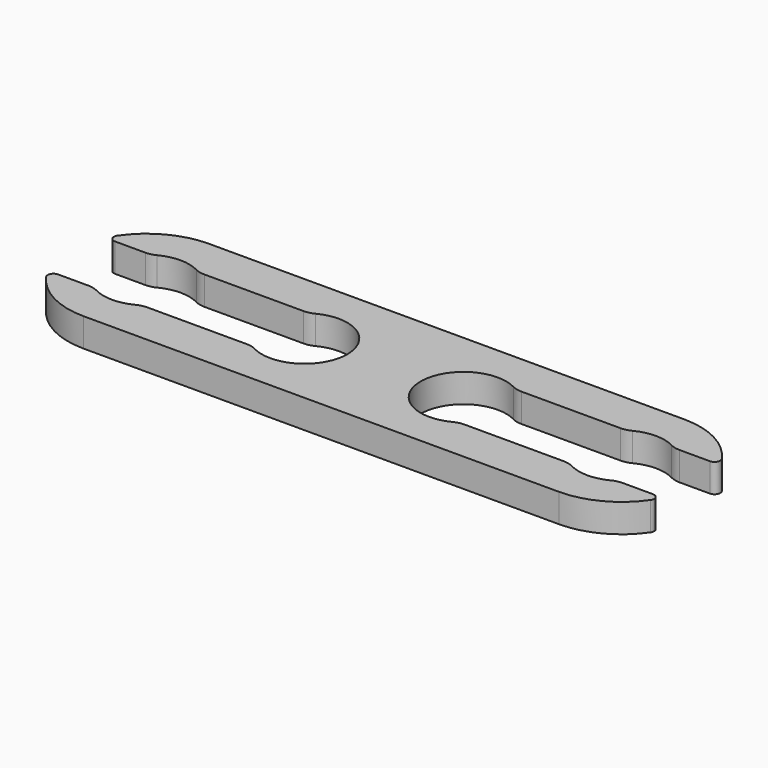
from build123d import *

# Parameters (mm, degrees)
F1_DEPTH = 2
F2_R     = 1.5
F3_R     = 0.4


with BuildPart() as f1:
    # F0 (on Top) → F1 (new body)
    with BuildSketch(Plane.XY):
        with BuildLine():
            ThreePointArc((-7.2316509448, 2.5), (-4.1547013841, 2.6433820369), (-2.5733385496, 0))
            ThreePointArc((-2.5733385496, 0), (-4.1547013841, -2.6433820369), (-7.2316509448, -2.5))
            Line((-7.2316509448, -2.5), (-11.7673134743, -2.5))
            ThreePointArc((-11.7673134743, -2.5), (-13.7940116366, -4.6904157598), (-16.6662929599, -5.5))
            Line((-16.6662929599, -5.5), (16.6662929599, -5.5))
            ThreePointArc((16.6662929599, -5.5), (13.7940116366, -4.6904157598), (11.7673134743, -2.5))
            Line((11.7673134743, -2.5), (7.2316509448, -2.5))
            ThreePointArc((7.2316509448, -2.5), (2.5733385496, 0), (7.2316509448, 2.5))
            Line((7.2316509448, 2.5), (11.7673134743, 2.5))
            ThreePointArc((11.7673134743, 2.5), (13.7940116366, 4.6904157598), (16.6662929599, 5.5))
            Line((16.6662929599, 5.5), (-16.6662929599, 5.5))
            ThreePointArc((-16.6662929599, 5.5), (-13.7940116366, 4.6904157598), (-11.7673134743, 2.5))
            Line((-11.7673134743, 2.5), (-7.2316509448, 2.5))
        make_face()
        with BuildLine():
            Line((-15.0079805647, 2.5), (-11.7673134743, 2.5))
            ThreePointArc((-11.7673134743, 2.5), (-13.7940116366, 4.6904157598), (-16.6662929599, 5.5))
            ThreePointArc((-16.6662929599, 5.5), (-19.5385742831, 4.6904157598), (-21.5652724454, 2.5))
            Line((-21.5652724454, 2.5), (-18.324605355, 2.5))
            ThreePointArc((-18.324605355, 2.5), (-16.6662929599, 3), (-15.0079805647, 2.5))
        make_face()
        with BuildLine():
            ThreePointArc((-16.6662929599, -5.5), (-13.7940116366, -4.6904157598), (-11.7673134743, -2.5))
            Line((-11.7673134743, -2.5), (-15.0079805647, -2.5))
            ThreePointArc((-15.0079805647, -2.5), (-16.6662929599, -3), (-18.324605355, -2.5))
            Line((-18.324605355, -2.5), (-21.5652724454, -2.5))
            ThreePointArc((-21.5652724454, -2.5), (-19.5385742831, -4.6904157598), (-16.6662929599, -5.5))
        make_face()
        with BuildLine():
            ThreePointArc((21.5652724454, 2.5), (19.5385742831, 4.6904157598), (16.6662929599, 5.5))
            ThreePointArc((16.6662929599, 5.5), (13.7940116366, 4.6904157598), (11.7673134743, 2.5))
            Line((11.7673134743, 2.5), (15.0079805647, 2.5))
            ThreePointArc((15.0079805647, 2.5), (16.6662929599, 3), (18.324605355, 2.5))
            Line((18.324605355, 2.5), (21.5652724454, 2.5))
        make_face()
        with BuildLine():
            ThreePointArc((11.7673134743, -2.5), (13.7940116366, -4.6904157598), (16.6662929599, -5.5))
            ThreePointArc((16.6662929599, -5.5), (19.5385742831, -4.6904157598), (21.5652724454, -2.5))
            Line((21.5652724454, -2.5), (18.324605355, -2.5))
            ThreePointArc((18.324605355, -2.5), (16.6662929599, -3), (15.0079805647, -2.5))
            Line((15.0079805647, -2.5), (11.7673134743, -2.5))
        make_face()
    extrude(amount=F1_DEPTH)

    # F2
    f2_edges = [f1.edges().sort_by_distance(p)[0] for p in [
        (-15.007981, 2.5, 1),
        (-18.324605, 2.5, 1),
        (-7.231651, 2.5, 1),
        (-18.324605, -2.5, 1),
        (-15.007981, -2.5, 1),
        (-7.231651, -2.5, 1),
        (7.231651, 2.5, 1),
        (18.324605, 2.5, 1),
        (15.007981, 2.5, 1),
        (7.231651, -2.5, 1),
        (15.007981, -2.5, 1),
        (18.324605, -2.5, 1),
    ]]
    fillet(f2_edges, radius=F2_R)

    # F3
    f3_edges = [f1.edges().sort_by_distance(p)[0] for p in [
        (21.565272, 2.5, 1),
        (21.565272, -2.5, 1),
        (-21.565272, 2.5, 1),
        (-21.565272, -2.5, 1),
    ]]
    fillet(f3_edges, radius=F3_R)


solid = f1.part
